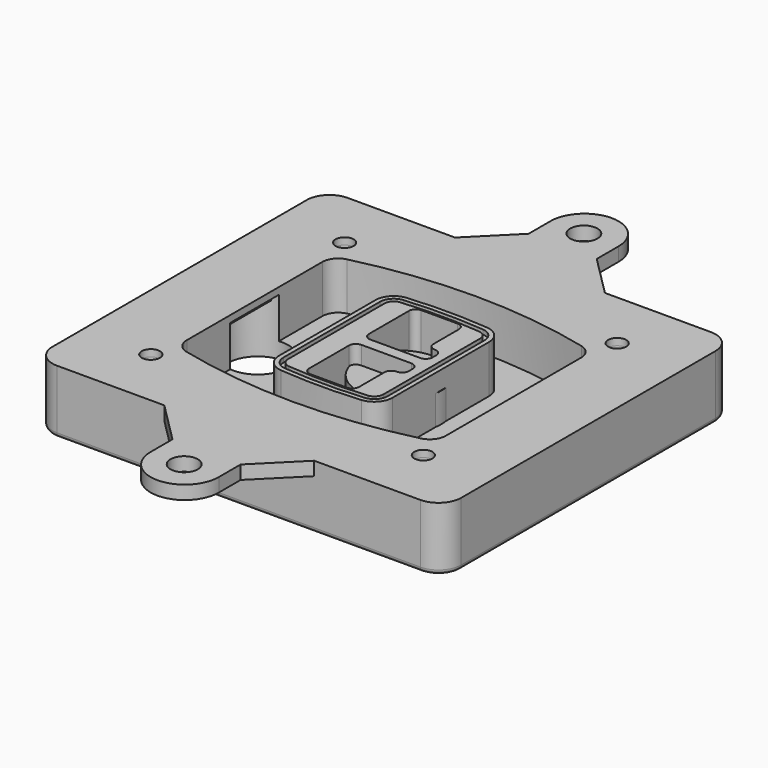
from build123d import *

# Parameters (mm, degrees)
F0_R      = 4
F1_DEPTH  = 25
F2_DEPTH  = 3
F3_DEPTH  = 18
F5_DEPTH  = 21
F6_DEPTH  = 2
F8_DEPTH  = 20
F9_DEPTH  = 16
F10_DEPTH = 25
F7_R      = 6
F7_R_2    = 4
F11_DEPTH = 6
F13_DEPTH = 9
F15_R     = 2
F16_R     = 6
F16_R_2   = 4
F17_DEPTH = 3


# Not quite as in the source:
# - a feature of the source that left no trace in its solid (it failed there, or was rolled back) is left out
# - a feature names something its author has since deleted; it is built from what else it names


with BuildPart() as f1:
    # F0 (on Top) → F1 (new body)
    with BuildSketch(Plane.XY):
        with BuildLine():
            ThreePointArc((-90, -70), (-87.0710678119, -77.0710678119), (-80, -80))
            Line((-80, -80), (80, -80))
            ThreePointArc((80, -80), (87.0710678119, -77.0710678119), (90, -70))
            Line((90, -70), (90, 70))
            ThreePointArc((90, 70), (87.0710678119, 77.0710678119), (80, 80))
            Line((80, 80), (-80, 80))
            ThreePointArc((-80, 80), (-87.0710678119, 77.0710678119), (-90, 70))
            Line((-90, 70), (-90, -70))
        make_face()
        with Locations((-60, -53.3333333333)):
            Circle(F0_R, mode=Mode.SUBTRACT)
        with Locations((60, -53.3333333333)):
            Circle(F0_R, mode=Mode.SUBTRACT)
        with Locations((-60, 53.3333333333)):
            Circle(F0_R, mode=Mode.SUBTRACT)
        with BuildLine():
            ThreePointArc((-64, 37.2990447398), (-61.0143011354, 45.9411029726), (-53.3306899286, 50.8970778549))
            ThreePointArc((-53.3306899286, 50.8970778549), (0, 57.3333333333), (53.3306899286, 50.8970778549))
            ThreePointArc((53.3306899286, 50.8970778549), (61.0143011354, 45.9411029726), (64, 37.2990447398))
            Line((64, 37.2990447398), (64, -37.2990447398))
            ThreePointArc((64, -37.2990447398), (61.0143011354, -45.9411029726), (53.3306899286, -50.8970778549))
            ThreePointArc((53.3306899286, -50.8970778549), (0, -57.3333333333), (-53.3306899286, -50.8970778549))
            ThreePointArc((-53.3306899286, -50.8970778549), (-61.0143011354, -45.9411029726), (-64, -37.2990447398))
            Line((-64, -37.2990447398), (-64, 37.2990447398))
        make_face(mode=Mode.SUBTRACT)
        with Locations((60, 53.3333333333)):
            Circle(F0_R, mode=Mode.SUBTRACT)
        with BuildLine():
            ThreePointArc((53.3306899286, 50.8970778549), (0, 57.3333333333), (-53.3306899286, 50.8970778549))
            ThreePointArc((-53.3306899286, 50.8970778549), (-61.0143011354, 45.9411029726), (-64, 37.2990447398))
            Line((-64, 37.2990447398), (-64, -37.2990447398))
            ThreePointArc((-64, -37.2990447398), (-61.0143011354, -45.9411029726), (-53.3306899286, -50.8970778549))
            ThreePointArc((-53.3306899286, -50.8970778549), (0, -57.3333333333), (53.3306899286, -50.8970778549))
            ThreePointArc((53.3306899286, -50.8970778549), (61.0143011354, -45.9411029726), (64, -37.2990447398))
            Line((64, -37.2990447398), (64, 37.2990447398))
            ThreePointArc((64, 37.2990447398), (61.0143011354, 45.9411029726), (53.3306899286, 50.8970778549))
        make_face()
        with BuildLine():
            Line((-60, -37.2990447398), (-60, 37.2990447398))
            ThreePointArc((-60, 37.2990447398), (-57.8673579538, 43.4719434775), (-52.3790642347, 47.0119255363))
            ThreePointArc((-52.3790642347, 47.0119255363), (0, 53.3333333333), (52.3790642347, 47.0119255363))
            ThreePointArc((52.3790642347, 47.0119255363), (57.8673579538, 43.4719434775), (60, 37.2990447398))
            Line((60, 37.2990447398), (60, -37.2990447398))
            ThreePointArc((60, -37.2990447398), (57.8673579538, -43.4719434775), (52.3790642347, -47.0119255363))
            ThreePointArc((52.3790642347, -47.0119255363), (0, -53.3333333333), (-52.3790642347, -47.0119255363))
            ThreePointArc((-52.3790642347, -47.0119255363), (-57.8673579538, -43.4719434775), (-60, -37.2990447398))
        make_face(mode=Mode.SUBTRACT)
        with BuildLine():
            ThreePointArc((-52.3790642347, 47.0119255363), (-57.8673579538, 43.4719434775), (-60, 37.2990447398))
            Line((-60, 37.2990447398), (-60, -37.2990447398))
            ThreePointArc((-60, -37.2990447398), (-57.8673579538, -43.4719434775), (-52.3790642347, -47.0119255363))
            ThreePointArc((-52.3790642347, -47.0119255363), (0, -53.3333333333), (52.3790642347, -47.0119255363))
            ThreePointArc((52.3790642347, -47.0119255363), (57.8673579538, -43.4719434775), (60, -37.2990447398))
            Line((60, -37.2990447398), (60, 37.2990447398))
            ThreePointArc((60, 37.2990447398), (57.8673579538, 43.4719434775), (52.3790642347, 47.0119255363))
            ThreePointArc((52.3790642347, 47.0119255363), (0, 53.3333333333), (-52.3790642347, 47.0119255363))
        make_face()
        with BuildLine():
            ThreePointArc((51.6653449643, 44.0980612973), (55.5071505677, 41.6200738562), (57, 37.2990447398))
            Line((57, 37.2990447398), (57, -37.2990447398))
            ThreePointArc((57, -37.2990447398), (55.5071505677, -41.6200738562), (51.6653449643, -44.0980612973))
            ThreePointArc((51.6653449643, -44.0980612973), (0, -50.3333333333), (-51.6653449643, -44.0980612973))
            ThreePointArc((-51.6653449643, -44.0980612973), (-55.5071505677, -41.6200738562), (-57, -37.2990447398))
            Line((-57, -37.2990447398), (-57, 37.2990447398))
            ThreePointArc((-57, 37.2990447398), (-55.5071505677, 41.6200738562), (-51.6653449643, 44.0980612973))
            ThreePointArc((-51.6653449643, 44.0980612973), (0, 50.3333333333), (51.6653449643, 44.0980612973))
        make_face(mode=Mode.SUBTRACT)
        with BuildLine():
            Line((57, -37.2990447398), (57, 37.2990447398))
            ThreePointArc((57, 37.2990447398), (55.5071505677, 41.6200738562), (51.6653449643, 44.0980612973))
            ThreePointArc((51.6653449643, 44.0980612973), (0, 50.3333333333), (-51.6653449643, 44.0980612973))
            ThreePointArc((-51.6653449643, 44.0980612973), (-55.5071505677, 41.6200738562), (-57, 37.2990447398))
            Line((-57, 37.2990447398), (-57, -37.2990447398))
            ThreePointArc((-57, -37.2990447398), (-55.5071505677, -41.6200738562), (-51.6653449643, -44.0980612973))
            ThreePointArc((-51.6653449643, -44.0980612973), (0, -50.3333333333), (51.6653449643, -44.0980612973))
            ThreePointArc((51.6653449643, -44.0980612973), (55.5071505677, -41.6200738562), (57, -37.2990447398))
        make_face()
    extrude(amount=-F1_DEPTH)

    # F0 (on Top) → F2 (join)
    with BuildSketch(Plane.XY):
        with BuildLine():
            ThreePointArc((-52.3790642347, 47.0119255363), (-57.8673579538, 43.4719434775), (-60, 37.2990447398))
            Line((-60, 37.2990447398), (-60, -37.2990447398))
            ThreePointArc((-60, -37.2990447398), (-57.8673579538, -43.4719434775), (-52.3790642347, -47.0119255363))
            ThreePointArc((-52.3790642347, -47.0119255363), (0, -53.3333333333), (52.3790642347, -47.0119255363))
            ThreePointArc((52.3790642347, -47.0119255363), (57.8673579538, -43.4719434775), (60, -37.2990447398))
            Line((60, -37.2990447398), (60, 37.2990447398))
            ThreePointArc((60, 37.2990447398), (57.8673579538, 43.4719434775), (52.3790642347, 47.0119255363))
            ThreePointArc((52.3790642347, 47.0119255363), (0, 53.3333333333), (-52.3790642347, 47.0119255363))
        make_face()
        with BuildLine():
            ThreePointArc((51.6653449643, 44.0980612973), (55.5071505677, 41.6200738562), (57, 37.2990447398))
            Line((57, 37.2990447398), (57, -37.2990447398))
            ThreePointArc((57, -37.2990447398), (55.5071505677, -41.6200738562), (51.6653449643, -44.0980612973))
            ThreePointArc((51.6653449643, -44.0980612973), (0, -50.3333333333), (-51.6653449643, -44.0980612973))
            ThreePointArc((-51.6653449643, -44.0980612973), (-55.5071505677, -41.6200738562), (-57, -37.2990447398))
            Line((-57, -37.2990447398), (-57, 37.2990447398))
            ThreePointArc((-57, 37.2990447398), (-55.5071505677, 41.6200738562), (-51.6653449643, 44.0980612973))
            ThreePointArc((-51.6653449643, 44.0980612973), (0, 50.3333333333), (51.6653449643, 44.0980612973))
        make_face(mode=Mode.SUBTRACT)
    extrude(amount=F2_DEPTH)

    # F0 (on Top) → F3 (cut)
    with BuildSketch(Plane.XY):
        with BuildLine():
            Line((57, -37.2990447398), (57, 37.2990447398))
            ThreePointArc((57, 37.2990447398), (55.5071505677, 41.6200738562), (51.6653449643, 44.0980612973))
            ThreePointArc((51.6653449643, 44.0980612973), (0, 50.3333333333), (-51.6653449643, 44.0980612973))
            ThreePointArc((-51.6653449643, 44.0980612973), (-55.5071505677, 41.6200738562), (-57, 37.2990447398))
            Line((-57, 37.2990447398), (-57, -37.2990447398))
            ThreePointArc((-57, -37.2990447398), (-55.5071505677, -41.6200738562), (-51.6653449643, -44.0980612973))
            ThreePointArc((-51.6653449643, -44.0980612973), (0, -50.3333333333), (51.6653449643, -44.0980612973))
            ThreePointArc((51.6653449643, -44.0980612973), (55.5071505677, -41.6200738562), (57, -37.2990447398))
        make_face()
    extrude(amount=-F3_DEPTH, mode=Mode.SUBTRACT)

    # F4 (on face) → F5 (join, through all)
    with BuildSketch(Plane.XY.offset(3)):
        with BuildLine():
            ThreePointArc((-25, -26.587695628), (-22.8992979869, -31.9912392117), (-17.7004291845, -34.5569740744))
            ThreePointArc((-17.7004291845, -34.5569740744), (0, -35.3333333333), (17.7004291845, -34.5569740744))
            ThreePointArc((17.7004291845, -34.5569740744), (22.8992979869, -31.9912392117), (25, -26.587695628))
            Line((25, -26.587695628), (25, 26.587695628))
            ThreePointArc((25, 26.587695628), (22.8992979869, 31.9912392117), (17.7004291845, 34.5569740744))
            ThreePointArc((17.7004291845, 34.5569740744), (0, 35.3333333333), (-17.7004291845, 34.5569740744))
            ThreePointArc((-17.7004291845, 34.5569740744), (-22.8992979869, 31.9912392117), (-25, 26.587695628))
            Line((-25, 26.587695628), (-25, -26.587695628))
        make_face()
        with BuildLine():
            ThreePointArc((17.5253218884, 32.5646544628), (21.4244734902, 30.6403533158), (23, 26.587695628))
            Line((23, 26.587695628), (23, -26.587695628))
            ThreePointArc((23, -26.587695628), (21.4244734902, -30.6403533158), (17.5253218884, -32.5646544628))
            ThreePointArc((17.5253218884, -32.5646544628), (0, -33.3333333333), (-17.5253218884, -32.5646544628))
            ThreePointArc((-17.5253218884, -32.5646544628), (-21.4244734902, -30.6403533158), (-23, -26.587695628))
            Line((-23, -26.587695628), (-23, 26.587695628))
            ThreePointArc((-23, 26.587695628), (-21.4244734902, 30.6403533158), (-17.5253218884, 32.5646544628))
            ThreePointArc((-17.5253218884, 32.5646544628), (0, 33.3333333333), (17.5253218884, 32.5646544628))
        make_face(mode=Mode.SUBTRACT)
        with BuildLine():
            Line((23, -26.587695628), (23, 26.587695628))
            ThreePointArc((23, 26.587695628), (21.4244734902, 30.6403533158), (17.5253218884, 32.5646544628))
            ThreePointArc((17.5253218884, 32.5646544628), (0, 33.3333333333), (-17.5253218884, 32.5646544628))
            ThreePointArc((-17.5253218884, 32.5646544628), (-21.4244734902, 30.6403533158), (-23, 26.587695628))
            Line((-23, 26.587695628), (-23, -26.587695628))
            ThreePointArc((-23, -26.587695628), (-21.4244734902, -30.6403533158), (-17.5253218884, -32.5646544628))
            ThreePointArc((-17.5253218884, -32.5646544628), (0, -33.3333333333), (17.5253218884, -32.5646544628))
            ThreePointArc((17.5253218884, -32.5646544628), (21.4244734902, -30.6403533158), (23, -26.587695628))
        make_face()
        with BuildLine():
            ThreePointArc((17.3502145923, 30.5723348512), (19.9496489934, 29.2894674198), (21, 26.587695628))
            Line((21, 26.587695628), (21, -26.587695628))
            ThreePointArc((21, -26.587695628), (19.9496489934, -29.2894674198), (17.3502145923, -30.5723348512))
            ThreePointArc((17.3502145923, -30.5723348512), (0, -31.3333333333), (-17.3502145923, -30.5723348512))
            ThreePointArc((-17.3502145923, -30.5723348512), (-19.9496489934, -29.2894674198), (-21, -26.587695628))
            Line((-21, -26.587695628), (-21, 26.587695628))
            ThreePointArc((-21, 26.587695628), (-19.9496489934, 29.2894674198), (-17.3502145923, 30.5723348512))
            ThreePointArc((-17.3502145923, 30.5723348512), (0, 31.3333333333), (17.3502145923, 30.5723348512))
        make_face(mode=Mode.SUBTRACT)
        with BuildLine():
            Line((21, -26.587695628), (21, 26.587695628))
            ThreePointArc((21, 26.587695628), (19.9496489934, 29.2894674198), (17.3502145923, 30.5723348512))
            ThreePointArc((17.3502145923, 30.5723348512), (0, 31.3333333333), (-17.3502145923, 30.5723348512))
            ThreePointArc((-17.3502145923, 30.5723348512), (-19.9496489934, 29.2894674198), (-21, 26.587695628))
            Line((-21, 26.587695628), (-21, -26.587695628))
            ThreePointArc((-21, -26.587695628), (-19.9496489934, -29.2894674198), (-17.3502145923, -30.5723348512))
            ThreePointArc((-17.3502145923, -30.5723348512), (0, -31.3333333333), (17.3502145923, -30.5723348512))
            ThreePointArc((17.3502145923, -30.5723348512), (19.9496489934, -29.2894674198), (21, -26.587695628))
        make_face()
        with BuildLine():
            Line((-8, -2.5), (14, -2.5))
            ThreePointArc((14, -2.5), (16.1213203436, -3.3786796564), (17, -5.5))
            Line((17, -5.5), (17, -7.5))
            ThreePointArc((17, -7.5), (16.1213203436, -9.6213203436), (14, -10.5))
            ThreePointArc((14, -10.5), (11.8786796564, -11.3786796564), (11, -13.5))
            Line((11, -13.5), (11, -27.5))
            ThreePointArc((11, -27.5), (10.1213203436, -29.6213203436), (8, -30.5))
            Line((8, -30.5), (-8, -30.5))
            ThreePointArc((-8, -30.5), (-10.1213203436, -29.6213203436), (-11, -27.5))
            Line((-11, -27.5), (-11, -5.5))
            ThreePointArc((-11, -5.5), (-10.1213203436, -3.3786796564), (-8, -2.5))
        make_face(mode=Mode.SUBTRACT)
        with BuildLine():
            ThreePointArc((-8, 2.5), (-10.1213203436, 3.3786796564), (-11, 5.5))
            Line((-11, 5.5), (-11, 27.5))
            ThreePointArc((-11, 27.5), (-10.1213203436, 29.6213203436), (-8, 30.5))
            Line((-8, 30.5), (8, 30.5))
            ThreePointArc((8, 30.5), (10.1213203436, 29.6213203436), (11, 27.5))
            Line((11, 27.5), (11, 13.5))
            ThreePointArc((11, 13.5), (11.8786796564, 11.3786796564), (14, 10.5))
            ThreePointArc((14, 10.5), (16.1213203436, 9.6213203436), (17, 7.5))
            Line((17, 7.5), (17, 5.5))
            ThreePointArc((17, 5.5), (16.1213203436, 3.3786796564), (14, 2.5))
            Line((14, 2.5), (-8, 2.5))
        make_face(mode=Mode.SUBTRACT)
    extrude(amount=-F5_DEPTH)

    # F4 (on face) → F6 (cut)
    with BuildSketch(Plane.XY.offset(3)):
        with BuildLine():
            Line((23, -26.587695628), (23, 26.587695628))
            ThreePointArc((23, 26.587695628), (21.4244734902, 30.6403533158), (17.5253218884, 32.5646544628))
            ThreePointArc((17.5253218884, 32.5646544628), (0, 33.3333333333), (-17.5253218884, 32.5646544628))
            ThreePointArc((-17.5253218884, 32.5646544628), (-21.4244734902, 30.6403533158), (-23, 26.587695628))
            Line((-23, 26.587695628), (-23, -26.587695628))
            ThreePointArc((-23, -26.587695628), (-21.4244734902, -30.6403533158), (-17.5253218884, -32.5646544628))
            ThreePointArc((-17.5253218884, -32.5646544628), (0, -33.3333333333), (17.5253218884, -32.5646544628))
            ThreePointArc((17.5253218884, -32.5646544628), (21.4244734902, -30.6403533158), (23, -26.587695628))
        make_face()
        with BuildLine():
            ThreePointArc((17.3502145923, 30.5723348512), (19.9496489934, 29.2894674198), (21, 26.587695628))
            Line((21, 26.587695628), (21, -26.587695628))
            ThreePointArc((21, -26.587695628), (19.9496489934, -29.2894674198), (17.3502145923, -30.5723348512))
            ThreePointArc((17.3502145923, -30.5723348512), (0, -31.3333333333), (-17.3502145923, -30.5723348512))
            ThreePointArc((-17.3502145923, -30.5723348512), (-19.9496489934, -29.2894674198), (-21, -26.587695628))
            Line((-21, -26.587695628), (-21, 26.587695628))
            ThreePointArc((-21, 26.587695628), (-19.9496489934, 29.2894674198), (-17.3502145923, 30.5723348512))
            ThreePointArc((-17.3502145923, 30.5723348512), (0, 31.3333333333), (17.3502145923, 30.5723348512))
        make_face(mode=Mode.SUBTRACT)
    extrude(amount=-F6_DEPTH, mode=Mode.SUBTRACT)

    # F7 (on face) → F8 (join)
    with BuildSketch(Plane(origin=(0, 0, -25), x_dir=(1, 0, 0), z_dir=(0, 0, -1))):
        with BuildLine():
            ThreePointArc((-6.71157564, 0), (6.7567035675, 13.4682792075), (20.224982775, 0))
            Line((20.224982775, 0), (25.224982775, 0))
            ThreePointArc((25.224982775, 0), (6.7567035675, 18.4682792075), (-11.71157564, 0))
            Line((-11.71157564, 0), (-6.71157564, 0))
        make_face()
        with BuildLine():
            Line((-6.71157564, 0), (20.224982775, 0))
            ThreePointArc((20.224982775, 0), (6.7567035675, 13.4682792075), (-6.71157564, 0))
        make_face()
        with BuildLine():
            ThreePointArc((-6.71157564, 0), (6.7567035675, -13.4682792075), (20.224982775, 0))
            Line((20.224982775, 0), (-6.71157564, 0))
        make_face()
        with BuildLine():
            Line((25.224982775, 0), (20.224982775, 0))
            ThreePointArc((20.224982775, 0), (6.7567035675, -13.4682792075), (-6.71157564, 0))
            Line((-6.71157564, 0), (-11.71157564, 0))
            ThreePointArc((-11.71157564, 0), (6.7567035675, -18.4682792075), (25.224982775, 0))
        make_face()
    extrude(amount=-F8_DEPTH)

    # F7 (on face) → F9 (cut)
    with BuildSketch(Plane(origin=(0, 0, -25), x_dir=(1, 0, 0), z_dir=(0, 0, -1))):
        with BuildLine():
            Line((-6.71157564, 0), (20.224982775, 0))
            ThreePointArc((20.224982775, 0), (6.7567035675, 13.4682792075), (-6.71157564, 0))
        make_face()
        with BuildLine():
            ThreePointArc((-6.71157564, 0), (6.7567035675, -13.4682792075), (20.224982775, 0))
            Line((20.224982775, 0), (-6.71157564, 0))
        make_face()
    extrude(amount=-F9_DEPTH, mode=Mode.SUBTRACT)

    # F7 (on face) → F10 (cut)
    with BuildSketch(Plane(origin=(0, 0, -25), x_dir=(1, 0, 0), z_dir=(0, 0, -1))):
        with BuildLine():
            Line((-69.0318229325, 0), (-42.0952645175, 0))
            ThreePointArc((-42.0952645175, 0), (-55.563543725, 13.4682792075), (-69.0318229325, 0))
        make_face()
        with BuildLine():
            ThreePointArc((-69.0318229325, 0), (-55.563543725, -13.4682792075), (-42.0952645175, 0))
            Line((-42.0952645175, 0), (-69.0318229325, 0))
        make_face()
    extrude(amount=-F10_DEPTH, mode=Mode.SUBTRACT)

    # F7 (on face) → F11 (cut)
    with BuildSketch(Plane(origin=(0, 0, -25), x_dir=(1, 0, 0), z_dir=(0, 0, -1))):
        with Locations((60, -53.3333333333)):
            Circle(F7_R)
        with Locations((60, -53.3333333333)):
            Circle(F7_R_2, mode=Mode.SUBTRACT)
        with Locations((-60, -53.3333333333)):
            Circle(F7_R)
        with Locations((-60, -53.3333333333)):
            Circle(F7_R_2, mode=Mode.SUBTRACT)
        with Locations((-60, 53.3333333333)):
            Circle(F7_R)
        with Locations((-60, 53.3333333333)):
            Circle(F7_R_2, mode=Mode.SUBTRACT)
        with Locations((60, 53.3333333333)):
            Circle(F7_R)
        with Locations((60, 53.3333333333)):
            Circle(F7_R_2, mode=Mode.SUBTRACT)
    extrude(amount=-F11_DEPTH, mode=Mode.SUBTRACT)

    # F12 (on face) → F13 (cut, through all)
    with BuildSketch(Plane(origin=(0, 0, -9), x_dir=(1, 0, 0), z_dir=(0, 0, -1))):
        with BuildLine():
            ThreePointArc((20.224982775, 0), (20.1663399806, 1.2554664788), (19.9909222755, 2.5))
            Line((19.9909222755, 2.5), (14, 2.5))
            ThreePointArc((14, 2.5), (16.1213203436, 3.3786796564), (17, 5.5))
            Line((17, 5.5), (17, 7.5))
            ThreePointArc((17, 7.5), (16.1213203436, 9.6213203436), (14, 10.5))
            ThreePointArc((14, 10.5), (12.1627255951, 11.1284134507), (11.0951631559, 12.750384826))
            ThreePointArc((11.0951631559, 12.750384826), (11.0476113807, 12.7664660322), (11, 12.7823698976))
            Line((11, 12.7823698976), (11, -12.7823698976))
            ThreePointArc((11, -12.7823698976), (11.0476113807, -12.7664660322), (11.0951631559, -12.750384826))
            ThreePointArc((11.0951631559, -12.750384826), (12.1627255951, -11.1284134507), (14, -10.5))
            ThreePointArc((14, -10.5), (16.1213203436, -9.6213203436), (17, -7.5))
            Line((17, -7.5), (17, -5.5))
            ThreePointArc((17, -5.5), (16.1213203436, -3.3786796564), (14, -2.5))
            Line((14, -2.5), (19.9909222755, -2.5))
            ThreePointArc((19.9909222755, -2.5), (20.1663399806, -1.2554664788), (20.224982775, 0))
        make_face()
    extrude(amount=F13_DEPTH, mode=Mode.SUBTRACT)

    # F15
    f15_edges = [f1.edges().sort_by_distance(p)[0] for p in [
        (0, -80, -25),
        (-87.071068, -77.071068, -25),
        (-90, 0, -25),
        (-87.071068, 77.071068, -25),
        (87.071068, -77.071068, -25),
        (0, 80, -25),
        (90, 0, -25),
        (87.071068, 77.071068, -25),
    ]]
    fillet(f15_edges, radius=F15_R)

    # F16 (on Top) → F17 (join, symmetric)
    with BuildSketch(Plane.XY):
        with BuildLine():
            Line((-14.7333178222, 98), (-32.7333178222, 80))
            Line((-32.7333178222, 80), (33.2666821778, 80))
            Line((33.2666821778, 80), (15.2666821778, 98))
            Line((15.2666821778, 98), (15.2666821778, 110))
            ThreePointArc((15.2666821778, 110), (0.2666821778, 125), (-14.7333178222, 110))
            Line((-14.7333178222, 110), (-14.7333178222, 98))
        make_face()
        with Locations((0, 110)):
            Circle(F16_R, mode=Mode.SUBTRACT)
        with BuildLine():
            Line((-32.7333178222, 80), (-80, 80))
            ThreePointArc((-80, 80), (-87.0710678119, 77.0710678119), (-90, 70))
            Line((-90, 70), (-90, -70))
            ThreePointArc((-90, -70), (-87.0710678119, -77.0710678119), (-80, -80))
            Line((-80, -80), (-32.7333178222, -80))
            Line((-32.7333178222, -80), (33.2666821778, -80))
            Line((33.2666821778, -80), (80, -80))
            ThreePointArc((80, -80), (87.0710678119, -77.0710678119), (90, -70))
            Line((90, -70), (90, 70))
            ThreePointArc((90, 70), (87.0710678119, 77.0710678119), (80, 80))
            Line((80, 80), (33.2666821778, 80))
            Line((33.2666821778, 80), (-32.7333178222, 80))
        make_face()
        with Locations((-60, -53.3333333333)):
            Circle(F16_R_2, mode=Mode.SUBTRACT)
        with Locations((60, -53.3333333333)):
            Circle(F16_R_2, mode=Mode.SUBTRACT)
        with Locations((-60, 53.3333333333)):
            Circle(F16_R_2, mode=Mode.SUBTRACT)
        with BuildLine():
            ThreePointArc((52.3790642347, -47.0119255363), (0, -53.3333333333), (-52.3790642347, -47.0119255363))
            ThreePointArc((-52.3790642347, -47.0119255363), (-57.8673579538, -43.4719434775), (-60, -37.2990447398))
            Line((-60, -37.2990447398), (-60, 37.2990447398))
            ThreePointArc((-60, 37.2990447398), (-57.8673579538, 43.4719434775), (-52.3790642347, 47.0119255363))
            ThreePointArc((-52.3790642347, 47.0119255363), (0, 53.3333333333), (52.3790642347, 47.0119255363))
            ThreePointArc((52.3790642347, 47.0119255363), (57.8673579538, 43.4719434775), (60, 37.2990447398))
            Line((60, 37.2990447398), (60, -37.2990447398))
            ThreePointArc((60, -37.2990447398), (57.8673579538, -43.4719434775), (52.3790642347, -47.0119255363))
        make_face(mode=Mode.SUBTRACT)
        with Locations((60, 53.3333333333)):
            Circle(F16_R_2, mode=Mode.SUBTRACT)
        with BuildLine():
            Line((33.2666821778, -80), (-32.7333178222, -80))
            Line((-32.7333178222, -80), (-14.7333178222, -98))
            Line((-14.7333178222, -98), (-14.7333178222, -110))
            ThreePointArc((-14.7333178222, -110), (0.2666821778, -125), (15.2666821778, -110))
            Line((15.2666821778, -110), (15.2666821778, -98))
            Line((15.2666821778, -98), (33.2666821778, -80))
        make_face()
        with Locations((0, -110)):
            Circle(F16_R, mode=Mode.SUBTRACT)
    extrude(amount=F17_DEPTH, both=True)


solid = f1.part
